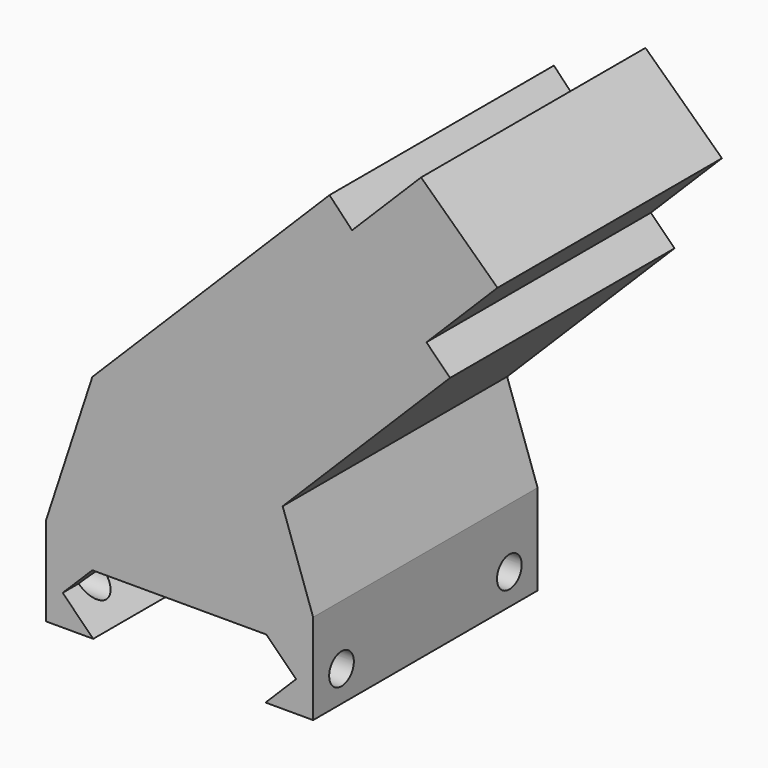
from build123d import *

# Parameters (mm, degrees)
F1_DEPTH = 25.4
F3_D     = 2.794
F3_DEPTH = 25.4
F3_TIP   = 0.8394022848
F4_D     = 2.794
F4_DEPTH = 25.4
F4_START = 10.1278152
F4_TIP   = 0.8394022848


# Not quite as in the source:
# - ends of sketch curves that miss each other by under 0.0002 mm in the source are joined
# - a feature names something its author has since deleted; it is built from what else it names


with BuildPart() as f1:
    # F0 (on Front) → F1 (new body)
    with BuildSketch(Plane.XZ):
        Polygon((11.0066256276, -6.5430273301), (8.240193387, -9.310965985), (12.5485987193, -9.310965985), (12.5485987193, -1.1086727812), (9.7906497979, 6.8444932552), (24.9488617122, 22.0027051695), (22.8072959293, 24.1442709524), (29.2404852808, 30.5774603039), (22.3196721338, 37.1254323684), (16.0729033236, 30.8786635582), (14.0302290969, 33.0205648235), (13.9806155776, 32.9709513042), (-7.4406042695, 11.5497314571), (-7.4406041338, 11.5466563515), (-7.4413635659, 11.5474157835), (-11.6305711889, -1.2286720797), (-11.6305711889, -9.3063699081), (-7.3613829189, -9.3063699081), (-10.1278151595, -6.5384312532), (-7.4425795762, -3.8636476732), (8.3167760077, -3.8636476732), align=None)
    extrude(amount=F1_DEPTH)

    # F3 (one way)
    with BuildSketch(Plane(origin=(0, 0, 0), x_dir=(0, 1, 0), z_dir=(-1, 0, 0))):
        with Locations((-22.1899207681, 6.5197679214), (-3.1917574815, 6.5197679214)):
            Circle(F3_D / 2)
    extrude(amount=-F3_DEPTH, mode=Mode.SUBTRACT)
    with Locations(Plane(origin=(0, 0, 0), x_dir=(0, 1, 0), z_dir=(-1, 0, 0))):
        with Locations((-22.1899207681, 6.5197679214), (-3.1917574815, 6.5197679214)):
            with Locations((0, 0, -(F3_DEPTH + F3_TIP / 2))):  # 118° drill point
                Cone(0, F3_D / 2, F3_TIP, mode=Mode.SUBTRACT)

    # F4
    # its depths count from where the whole tool has entered the part; down to there all is cleared
    with Locations(Plane.YZ.offset(-F4_START)):
        with Locations((-3.1917574815, -6.5197679214), (-22.1899207681, -6.5197679214)):
            Hole(F4_D / 2, depth=F4_DEPTH)
            with Locations((0, 0, -(F4_DEPTH + F4_TIP / 2))):  # 118° drill point
                Cone(0, F4_D / 2, F4_TIP, mode=Mode.SUBTRACT)


solid = f1.part
